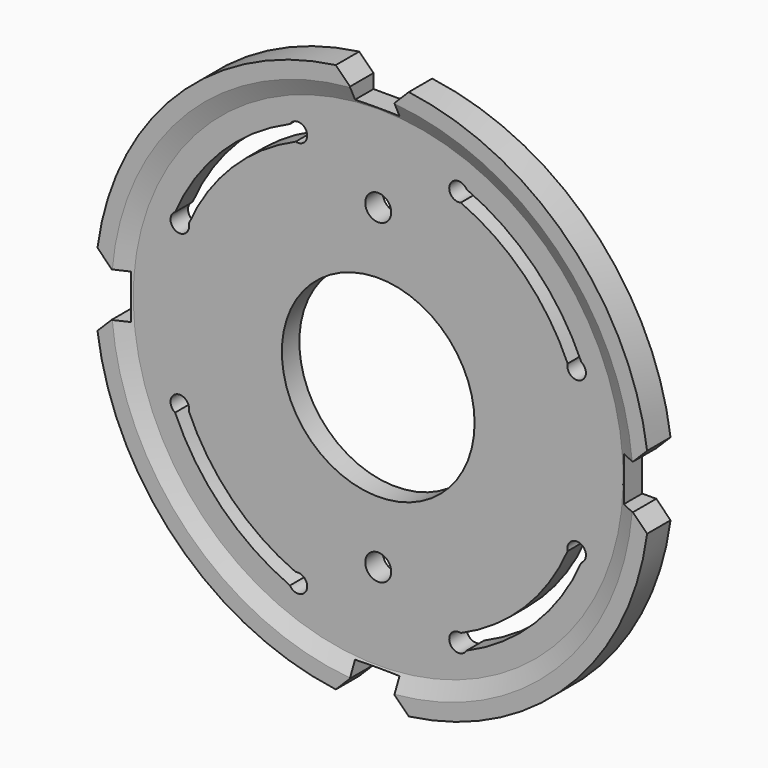
from build123d import *

# Parameters (mm, degrees)
F0_R     = 74.8
F0_R_2   = 3.5
F0_R_3   = 26
F1_DEPTH = 7.9
F2_DEPTH = 7.9
F3_R     = 66.1
F3_R_2   = 3.5
F3_R_3   = 26
F4_DEPTH = 2
F8_DEPTH = 5.9
F9_DEPTH = 2


# Not quite as in the source:
# - a feature names something its author has since deleted; it is built from what else it names


with BuildPart() as f1:
    # F0 (on Front) → F1 (new body)
    with BuildSketch(Plane.XZ):
        Circle(F0_R)
        with BuildLine():
            ThreePointArc((-23.816128087, -54.7983078474), (-42.2496301759, -42.2496301759), (-54.7983078474, -23.816128087))
            ThreePointArc((-54.7983078474, -23.816128087), (-54.50218665, -19.353932752), (-51.1097752784, -22.2677652896))
            ThreePointArc((-51.1097752784, -22.2677652896), (-39.4212030512, -39.4212030512), (-22.2677652896, -51.1097752784))
            ThreePointArc((-22.2677652896, -51.1097752784), (-19.353932752, -54.50218665), (-23.816128087, -54.7983078474))
        make_face(mode=Mode.SUBTRACT)
        with Locations((0, -42.7)):
            Circle(F0_R_2, mode=Mode.SUBTRACT)
        Circle(F0_R_3, mode=Mode.SUBTRACT)
        with BuildLine():
            ThreePointArc((54.7983078474, -23.816128087), (42.2496301759, -42.2496301759), (23.816128087, -54.7983078474))
            ThreePointArc((23.816128087, -54.7983078474), (19.353932752, -54.50218665), (22.2677652896, -51.1097752784))
            ThreePointArc((22.2677652896, -51.1097752784), (39.4212030512, -39.4212030512), (51.1097752784, -22.2677652896))
            ThreePointArc((51.1097752784, -22.2677652896), (54.50218665, -19.353932752), (54.7983078474, -23.816128087))
        make_face(mode=Mode.SUBTRACT)
        with BuildLine():
            ThreePointArc((-54.7983078474, 23.816128087), (-42.2496301759, 42.2496301759), (-23.816128087, 54.7983078474))
            ThreePointArc((-23.816128087, 54.7983078474), (-19.353932752, 54.50218665), (-22.2677652896, 51.1097752784))
            ThreePointArc((-22.2677652896, 51.1097752784), (-39.4212030512, 39.4212030512), (-51.1097752784, 22.2677652896))
            ThreePointArc((-51.1097752784, 22.2677652896), (-54.50218665, 19.353932752), (-54.7983078474, 23.816128087))
        make_face(mode=Mode.SUBTRACT)
        with Locations((0, 42.7)):
            Circle(F0_R_2, mode=Mode.SUBTRACT)
        with BuildLine():
            ThreePointArc((54.7983078474, 23.816128087), (54.50218665, 19.353932752), (51.1097752784, 22.2677652896))
            ThreePointArc((51.1097752784, 22.2677652896), (39.4212030512, 39.4212030512), (22.2677652896, 51.1097752784))
            ThreePointArc((22.2677652896, 51.1097752784), (19.353932752, 54.50218665), (23.816128087, 54.7983078474))
            ThreePointArc((23.816128087, 54.7983078474), (42.2496301759, 42.2496301759), (54.7983078474, 23.816128087))
        make_face(mode=Mode.SUBTRACT)
        Circle(F0_R_3)
    extrude(amount=-F1_DEPTH)

    # F0 (on Front) → F2 (cut)
    with BuildSketch(Plane.XZ):
        Circle(F0_R_3)
    extrude(amount=-F2_DEPTH, mode=Mode.SUBTRACT)

    # F3 (on face) → F4 (cut)
    with BuildSketch(Plane.XZ):
        Circle(F3_R)
        with BuildLine():
            ThreePointArc((-22.2677652896, -51.1097752784), (-19.353932752, -54.50218665), (-23.816128087, -54.7983078474))
            ThreePointArc((-23.816128087, -54.7983078474), (-42.2496301759, -42.2496301759), (-54.7983078474, -23.816128087))
            ThreePointArc((-54.7983078474, -23.816128087), (-54.50218665, -19.353932752), (-51.1097752784, -22.2677652896))
            ThreePointArc((-51.1097752784, -22.2677652896), (-39.4212030512, -39.4212030512), (-22.2677652896, -51.1097752784))
        make_face(mode=Mode.SUBTRACT)
        with Locations((0, -42.7)):
            Circle(F3_R_2, mode=Mode.SUBTRACT)
        Circle(F3_R_3, mode=Mode.SUBTRACT)
        with BuildLine():
            ThreePointArc((51.1097752784, -22.2677652896), (54.50218665, -19.353932752), (54.7983078474, -23.816128087))
            ThreePointArc((54.7983078474, -23.816128087), (42.2496301759, -42.2496301759), (23.816128087, -54.7983078474))
            ThreePointArc((23.816128087, -54.7983078474), (19.353932752, -54.50218665), (22.2677652896, -51.1097752784))
            ThreePointArc((22.2677652896, -51.1097752784), (39.4212030512, -39.4212030512), (51.1097752784, -22.2677652896))
        make_face(mode=Mode.SUBTRACT)
        with BuildLine():
            ThreePointArc((-51.1097752784, 22.2677652896), (-54.50218665, 19.353932752), (-54.7983078474, 23.816128087))
            ThreePointArc((-54.7983078474, 23.816128087), (-42.2496301759, 42.2496301759), (-23.816128087, 54.7983078474))
            ThreePointArc((-23.816128087, 54.7983078474), (-19.353932752, 54.50218665), (-22.2677652896, 51.1097752784))
            ThreePointArc((-22.2677652896, 51.1097752784), (-39.4212030512, 39.4212030512), (-51.1097752784, 22.2677652896))
        make_face(mode=Mode.SUBTRACT)
        with Locations((0, 42.7)):
            Circle(F3_R_2, mode=Mode.SUBTRACT)
        with BuildLine():
            ThreePointArc((23.816128087, 54.7983078474), (42.2496301759, 42.2496301759), (54.7983078474, 23.816128087))
            ThreePointArc((54.7983078474, 23.816128087), (54.50218665, 19.353932752), (51.1097752784, 22.2677652896))
            ThreePointArc((51.1097752784, 22.2677652896), (39.4212030512, 39.4212030512), (22.2677652896, 51.1097752784))
            ThreePointArc((22.2677652896, 51.1097752784), (19.353932752, 54.50218665), (23.816128087, 54.7983078474))
        make_face(mode=Mode.SUBTRACT)
    extrude(amount=-F4_DEPTH, mode=Mode.SUBTRACT)

    # F5 (on Right) → F6 (revolve, cut)
    with BuildSketch(Plane.YZ):
        Polygon((-1.7160152132, 0), (2, 0), (2, 66.1), (-1.7160152132, 74.0690203414), align=None)
    revolve(axis=Axis((0, 0.1419923934, 0), (0, 1, 0)), mode=Mode.SUBTRACT)

    # F7 (on face) → F8 (cut)
    with BuildSketch(Plane.XZ.offset(-2)):
        Polygon((-6, 70.3), (-6, 66.5), (6, 66.5), (6, 70.3), (12.4951375847, 76.7951375847), (-12.3430622144, 76.6430622144), align=None)
        Polygon((-66.5, 6), (-70.3, 6), (-76.7951375847, 12.4951375847), (-76.6430622144, -12.3430622144), (-70.3, -6), (-66.5, -6), align=None)
        Polygon((-6, -66.5), (-6, -70.3), (-12.4951375847, -76.7951375847), (12.3430622144, -76.6430622144), (6, -70.3), (6, -66.5), align=None)
        Polygon((66.5, -6), (70.3, -6), (76.7951375847, -12.4951375847), (76.6430622144, 12.3430622144), (70.3, 6), (66.5, 6), align=None)
    extrude(amount=-F8_DEPTH, mode=Mode.SUBTRACT)

    # F9 (cut): faces of the model
    f9_faces = [f1.faces().sort_by_distance(p)[0] for p in [
        (0, 2, 70.9549233508),
        (0, 2, -70.9549233508),
        (-70.9549233508, 2, 0),
        (70.9549233508, 2, 0),
    ]]
    extrude(f9_faces, amount=-F9_DEPTH, mode=Mode.SUBTRACT)


solid = f1.part
